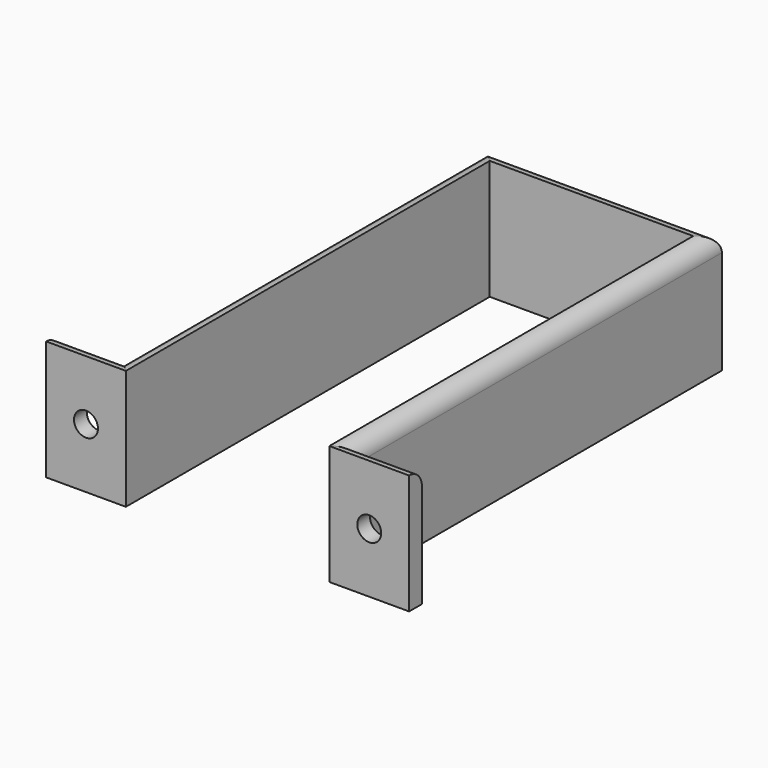
from build123d import *

# Parameters (mm, degrees)
F1_DEPTH = 15
F2_R     = 1.5
F3_DEPTH = 2
F4_R     = 1.99999


# Not quite as in the source:
# - a fillet or chamfer is up to 0.001 mm smaller than in the source, because OpenCascade refuses the exact size


with BuildPart() as f1:
    # F0 (on Top) → F1 (new body)
    with BuildSketch(Plane.XY):
        Polygon((-22.75, 2), (-22.75, 0), (-12.75, 0), (-12.75, 57), (0, 57), (12.75, 57), (12.75, 0), (22.75, 0), (22.75, 2), (14.75, 2), (14.75, 59), (0, 59), (-14.75, 59), (-14.75, 2), align=None)
    extrude(amount=F1_DEPTH)

    # F2 (on Front) → F3 (cut)
    with BuildSketch(Plane.XZ):
        with Locations((-17.75, 7.5)):
            Circle(F2_R)
        with Locations((17.75, 7.5)):
            Circle(F2_R)
    extrude(amount=-F3_DEPTH, mode=Mode.SUBTRACT)

    # F4 (radius 2 in the source; OpenCascade refuses exactly that, so slightly less here)
    f4_edges = [f1.edges().sort_by_distance(p)[0] for p in [
        (-14.75, 30.5, 15),
        (0, 59, 15),
        (14.75, 30.5, 15),
        (18.75, 2, 15),
        (-18.75, 2, 15),
    ]]
    fillet(f4_edges, radius=F4_R)


solid = f1.part
